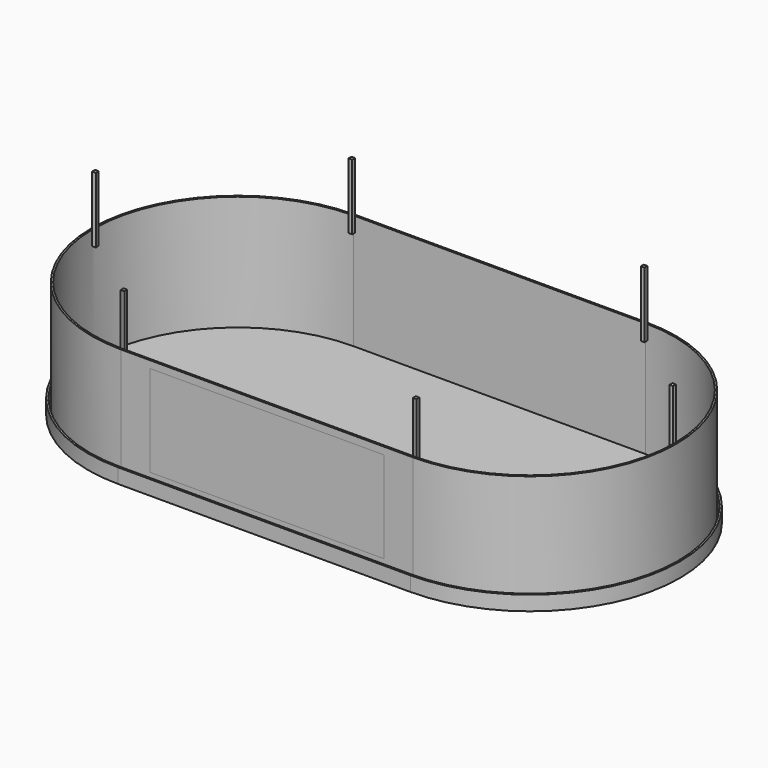
from build123d import *

# Parameters (mm, degrees)
F1_DEPTH       = 203.2
F2_T           = -3.175
F4_W           = 406.4
F4_H           = 158.75
F5_DEPTH       = 25.4
F6_W           = 406.4
F6_H           = 158.75
F7_DEPTH       = 3.175
F10_DEPTH      = 25.4
F11_T          = -3.175
F14_DEPTH      = 25.4
F14_DEPTH_BACK = 88.9


with BuildPart() as f1:
    # F0 (on Top) → F1 (new body)
    with BuildSketch(Plane.XY):
        with BuildLine():
            Line((-508, -254), (0, -254))
            ThreePointArc((0, -254), (254, 0), (0, 254))
            Line((0, 254), (-508, 254))
            ThreePointArc((-508, 254), (-762, 0), (-508, -254))
        make_face()
    extrude(amount=F1_DEPTH)

    # F2
    f2_openings = [f1.faces().sort_by_distance(p)[0] for p in [
        (-254, 0, 203.2),
    ]]
    offset(amount=F2_T, openings=f2_openings)

    # F4 (on offset) → F5 (cut)
    with BuildSketch(Plane.XZ.offset(254)):
        with Locations((-254, 111.125)):
            Rectangle(F4_W, F4_H)
    extrude(amount=-F5_DEPTH, mode=Mode.SUBTRACT)

    # F13 (on offset) → F14 (join, two sides)
    with BuildSketch(Plane.XY.offset(203.2)) as f14_sk:
        with BuildLine():
            ThreePointArc((250.8049042583, -3.175), (250.825, 0), (250.8049042583, 3.175))
            Line((250.8049042583, 3.175), (244.8118613124, 3.175))
            Line((244.8118613124, 3.175), (244.8118613124, -3.175))
            Line((244.8118613124, -3.175), (250.8049042583, -3.175))
        make_face()
        with BuildLine():
            Line((0, 250.825), (-3.175, 250.825))
            Line((-3.175, 250.825), (-3.175, 244.4750070572))
            Line((-3.175, 244.4750070572), (0, 244.4750070572))
            Line((0, 244.4750070572), (3.175, 244.4750070572))
            Line((3.175, 244.4750070572), (3.175, 250.8049042583))
            ThreePointArc((3.175, 250.8049042583), (1.587531798, 250.8199760143), (0, 250.825))
        make_face()
        with BuildLine():
            Line((-504.825, 250.825), (-508, 250.825))
            ThreePointArc((-508, 250.825), (-509.587531798, 250.8199760143), (-511.175, 250.8049042583))
            Line((-511.175, 250.8049042583), (-511.175, 244.4750070572))
            Line((-511.175, 244.4750070572), (-508, 244.4750070572))
            Line((-508, 244.4750070572), (-504.825, 244.4750070572))
            Line((-504.825, 244.4750070572), (-504.825, 250.825))
        make_face()
        with BuildLine():
            Line((-752.475, 3.175), (-758.8049042583, 3.175))
            ThreePointArc((-758.8049042583, 3.175), (-758.825, 0), (-758.8049042583, -3.175))
            Line((-758.8049042583, -3.175), (-752.475, -3.175))
            Line((-752.475, -3.175), (-752.475, 0))
            Line((-752.475, 0), (-752.475, 3.175))
        make_face()
        with BuildLine():
            Line((-511.175, -244.4750070572), (-511.175, -250.8049042583))
            ThreePointArc((-511.175, -250.8049042583), (-509.587531798, -250.8199760143), (-508, -250.825))
            Line((-508, -250.825), (-504.825, -250.825))
            Line((-504.825, -250.825), (-504.825, -244.4750070572))
            Line((-504.825, -244.4750070572), (-508, -244.4750070572))
            Line((-508, -244.4750070572), (-511.175, -244.4750070572))
        make_face()
        with BuildLine():
            Line((-3.175, -244.4750070572), (-3.175, -250.825))
            Line((-3.175, -250.825), (0, -250.825))
            ThreePointArc((0, -250.825), (1.587531798, -250.8199760143), (3.175, -250.8049042583))
            Line((3.175, -250.8049042583), (3.175, -244.4750070572))
            Line((3.175, -244.4750070572), (0, -244.4750070572))
            Line((0, -244.4750070572), (-3.175, -244.4750070572))
        make_face()
    extrude(amount=-F14_DEPTH)
    extrude(f14_sk.sketch, amount=F14_DEPTH_BACK)


with BuildPart() as f7:
    # F6 (on offset) → F7 (new body)
    with BuildSketch(Plane.XZ.offset(254)):
        with Locations((-254, 111.125)):
            Rectangle(F6_W, F6_H)
    extrude(amount=-F7_DEPTH)


with BuildPart() as f10:
    # F9 (on offset) → F10 (new body)
    with BuildSketch(Plane(origin=(0, 0, 0), x_dir=(1, 0, 0), z_dir=(0, 0, -1))):
        with BuildLine():
            ThreePointArc((-508, 260.3500051498), (-768.3500051498, 0), (-508, -260.3500051498))
            Line((-508, -260.3500051498), (0, -260.3500051498))
            ThreePointArc((0, -260.3500051498), (260.3500051498, 0), (0, 260.3500051498))
            Line((0, 260.3500051498), (-508, 260.3500051498))
        make_face()
    extrude(amount=-F10_DEPTH)

    # F11
    f11_openings = [f10.faces().sort_by_distance(p)[0] for p in [
        (-254, 0, 25.4),
    ]]
    offset(amount=F11_T, openings=f11_openings)


solid = Compound([f1.part, f7.part, f10.part])
